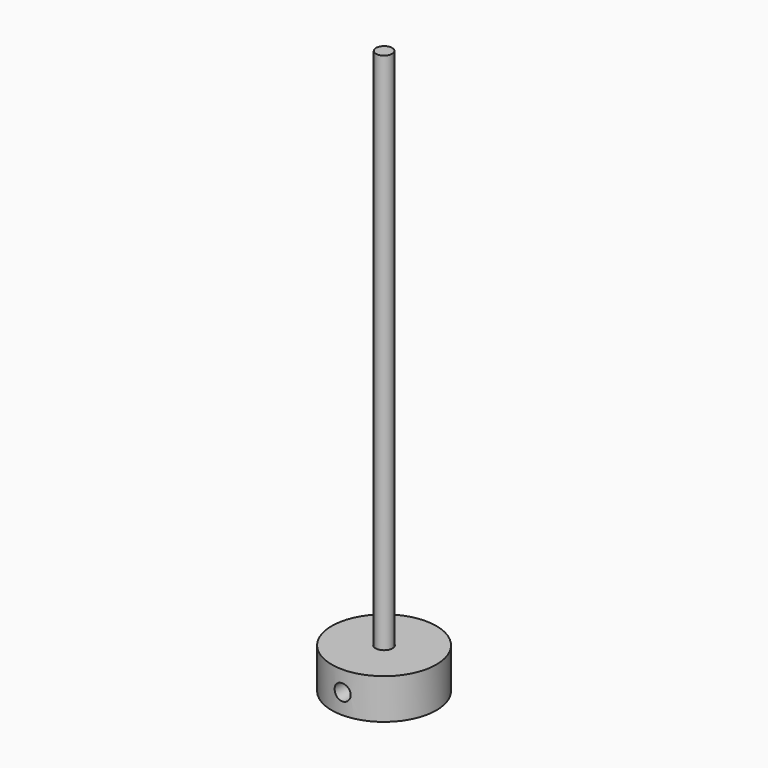
from build123d import *

# Parameters (mm, degrees)
F0_R     = 1
F1_DEPTH = 70
F3_DEPTH = 12.5
F4_R     = 6.5
F4_R_2   = 1.05
F5_DEPTH = 5
F6_R     = 1
F7_DEPTH = 12.5


with BuildPart() as f1:
    # F0 (on Top) → F1 (new body)
    with BuildSketch(Plane.XY):
        Circle(F0_R)
    extrude(amount=F1_DEPTH)

    # F2 (on Front) → F3 (cut, symmetric)
    with BuildSketch(Plane.XZ):
        Polygon((1.154513564, 3.092951607), (0.1861076162, 0), (1.154513564, 0), align=None)
        Polygon((-1.154513564, 0), (-0.1861076162, 0), (-1.154513564, 3.092951607), align=None)
    extrude(amount=F3_DEPTH, both=True, mode=Mode.SUBTRACT)


with BuildPart() as f5:
    # F4 (on Top) → F5 (new body)
    with BuildSketch(Plane.XY):
        Circle(F4_R)
        Circle(F4_R_2, mode=Mode.SUBTRACT)
    extrude(amount=F5_DEPTH)

    # F6 (on Front) → F7 (cut, symmetric)
    with BuildSketch(Plane.XZ):
        with Locations((0, 2.5)):
            Circle(F6_R)
    extrude(amount=F7_DEPTH, both=True, mode=Mode.SUBTRACT)


solid = Compound([f1.part, f5.part])
